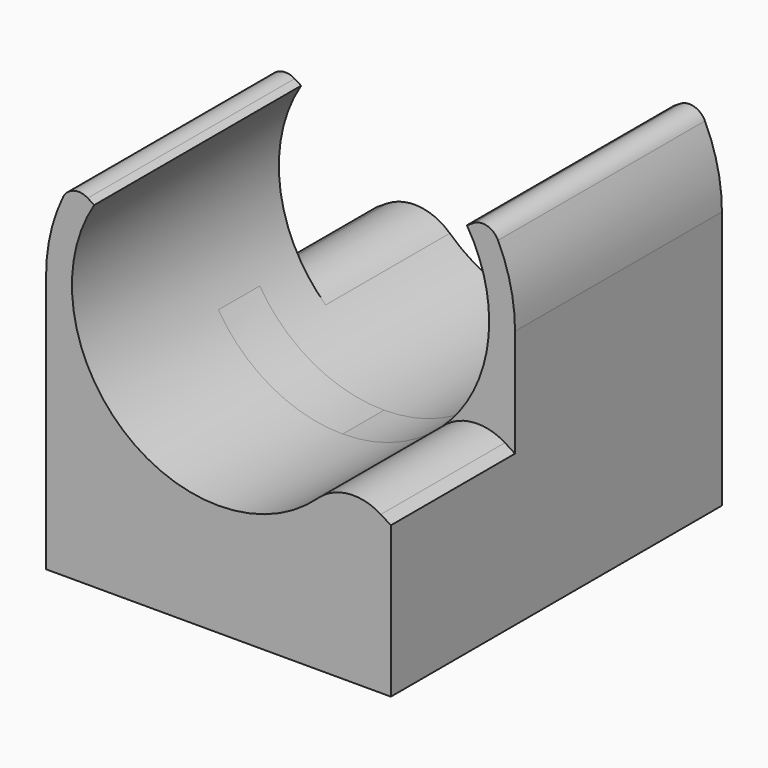
from build123d import *

# Parameters (mm, degrees)
F1_DEPTH      = 12
F1_DEPTH_BACK = 3
F2_DEPTH      = 12
F2_DEPTH_BACK = 3
F3_T1_DEPTH   = 15.504504139
F3_T3_DEPTH   = 15.504504139
F4_R          = 1
F5_DEPTH      = 5


# Not quite as in the source:
# - a fillet or chamfer that OpenCascade refuses, or shapes differently, is made with other operations: its cross-section is extruded or revolved along the edge and cut away or added


with BuildPart() as f1:
    # F0 (on Front) → F1 (new body, two sides)
    with BuildSketch(Plane.XZ) as f1_sk:
        with BuildLine():
            Line((10, -6.2486935191), (8.4804809616, -5.2991926423))
            ThreePointArc((8.4804809616, -5.2991926423), (4.8480962025, -8.7461970714), (0, -10))
            Line((0, -10), (10, -10))
            Line((10, -10), (10, -6.2486935191))
        make_face()
        with BuildLine():
            Line((-10, -10), (0, -10))
            ThreePointArc((0, -10), (-4.8480962025, -8.7461970714), (-8.4804809616, -5.2991926423))
            Line((-8.4804809616, -5.2991926423), (-10, -6.2486935191))
            Line((-10, -6.2486935191), (-10, -10))
        make_face()
        with BuildLine():
            Line((8.4804809616, -5.2991926423), (7.2084088173, -4.504313746))
            ThreePointArc((7.2084088173, -4.504313746), (4.1208817721, -7.4342675107), (0, -8.5))
            Line((0, -8.5), (0, -10))
            ThreePointArc((0, -10), (4.8480962025, -8.7461970714), (8.4804809616, -5.2991926423))
        make_face()
        with BuildLine():
            Line((0, -10), (0, -8.5))
            ThreePointArc((0, -8.5), (-4.1208817721, -7.4342675107), (-7.2084088173, -4.504313746))
            Line((-7.2084088173, -4.504313746), (-8.4804809616, -5.2991926423))
            ThreePointArc((-8.4804809616, -5.2991926423), (-4.8480962025, -8.7461970714), (0, -10))
        make_face()
        with BuildLine():
            ThreePointArc((-7.2084088173, -4.504313746), (-8.5, 0), (-7.2084088173, 4.504313746))
            Line((-7.2084088173, 4.504313746), (-8.4804809616, 5.2991926423))
            ThreePointArc((-8.4804809616, 5.2991926423), (-9.6126169594, 2.7563735582), (-10, 0))
            ThreePointArc((-10, 0), (-9.6126169594, -2.7563735582), (-8.4804809616, -5.2991926423))
            Line((-8.4804809616, -5.2991926423), (-7.2084088173, -4.504313746))
        make_face()
        with BuildLine():
            Line((-10, -6.2486935191), (-8.4804809616, -5.2991926423))
            ThreePointArc((-8.4804809616, -5.2991926423), (-9.6126169594, -2.7563735582), (-10, 0))
            Line((-10, 0), (-10, -6.2486935191))
        make_face()
    extrude(amount=F1_DEPTH)
    extrude(f1_sk.sketch, amount=-F1_DEPTH_BACK)

    # F0 (on Front) → F2 (join, two sides)
    with BuildSketch(Plane.XZ) as f2_sk:
        with BuildLine():
            Line((-10, -10), (0, -10))
            ThreePointArc((0, -10), (-4.8480962025, -8.7461970714), (-8.4804809616, -5.2991926423))
            Line((-8.4804809616, -5.2991926423), (-10, -6.2486935191))
            Line((-10, -6.2486935191), (-10, -10))
        make_face()
        with BuildLine():
            Line((8.4804809616, -5.2991926423), (7.2084088173, -4.504313746))
            ThreePointArc((7.2084088173, -4.504313746), (4.1208817721, -7.4342675107), (0, -8.5))
            Line((0, -8.5), (0, -10))
            ThreePointArc((0, -10), (4.8480962025, -8.7461970714), (8.4804809616, -5.2991926423))
        make_face()
        with BuildLine():
            Line((0, -10), (0, -8.5))
            ThreePointArc((0, -8.5), (-4.1208817721, -7.4342675107), (-7.2084088173, -4.504313746))
            Line((-7.2084088173, -4.504313746), (-8.4804809616, -5.2991926423))
            ThreePointArc((-8.4804809616, -5.2991926423), (-4.8480962025, -8.7461970714), (0, -10))
        make_face()
        with BuildLine():
            Line((10, -6.2486935191), (8.4804809616, -5.2991926423))
            ThreePointArc((8.4804809616, -5.2991926423), (4.8480962025, -8.7461970714), (0, -10))
            Line((0, -10), (10, -10))
            Line((10, -10), (10, -6.2486935191))
        make_face()
        with BuildLine():
            ThreePointArc((7.2084088173, 4.504313746), (8.1707244155, 2.3429175244), (8.5, 0))
            ThreePointArc((8.5, 0), (8.1707244155, -2.3429175244), (7.2084088173, -4.504313746))
            Line((7.2084088173, -4.504313746), (8.4804809616, -5.2991926423))
            ThreePointArc((8.4804809616, -5.2991926423), (9.6126169594, -2.7563735582), (10, 0))
            ThreePointArc((10, 0), (9.6126169594, 2.7563735582), (8.4804809616, 5.2991926423))
            Line((8.4804809616, 5.2991926423), (7.2084088173, 4.504313746))
        make_face()
        with BuildLine():
            ThreePointArc((10, 0), (9.6126169594, -2.7563735582), (8.4804809616, -5.2991926423))
            Line((8.4804809616, -5.2991926423), (10, -6.2486935191))
            Line((10, -6.2486935191), (10, 0))
        make_face()
    extrude(amount=-F2_DEPTH)
    extrude(f2_sk.sketch, amount=F2_DEPTH_BACK)

    # F3: fillet of radius 3 on 2 edges, made by hand

    # F3_s2 → F3_t1 (cut)
    with BuildSketch(Plane.XZ.offset(-18.504504139)):
        with BuildLine():
            ThreePointArc((-9.4148617579, -5.883058565), (-7.5407373956, -5.4407106546), (-5.783772496, -6.2288021091))
            ThreePointArc((-5.783772496, -6.2288021091), (-6.5530648439, -5.413625509), (-7.2084088173, -4.504313746))
            Line((-7.2084088173, -4.504313746), (-9.4148617579, -5.883058565))
        make_face()
    extrude(amount=F3_T1_DEPTH, mode=Mode.SUBTRACT)

    # F3_s4 → F3_t3 (cut)
    with BuildSketch(Plane.XZ.offset(3)):
        with BuildLine():
            ThreePointArc((5.783772496, -6.2288021091), (7.5407373956, -5.4407106546), (9.4148617579, -5.883058565))
            Line((9.4148617579, -5.883058565), (7.2084088173, -4.504313746))
            ThreePointArc((7.2084088173, -4.504313746), (6.5530648439, -5.413625509), (5.783772496, -6.2288021091))
        make_face()
    extrude(amount=F3_T3_DEPTH, mode=Mode.SUBTRACT)

    # F4
    f4_edges = [f1.edges().sort_by_distance(p)[0] for p in [
        (8.480481, 4.5, 5.299193),
        (-8.480481, -4.5, 5.299193),
    ]]
    fillet(f4_edges, radius=F4_R)

    # F5 (add): a face of the model
    f5_faces = [f1.faces().sort_by_distance(p)[0] for p in [
        (0, 0, -10),
    ]]
    extrude(f5_faces, amount=F5_DEPTH)


solid = f1.part
